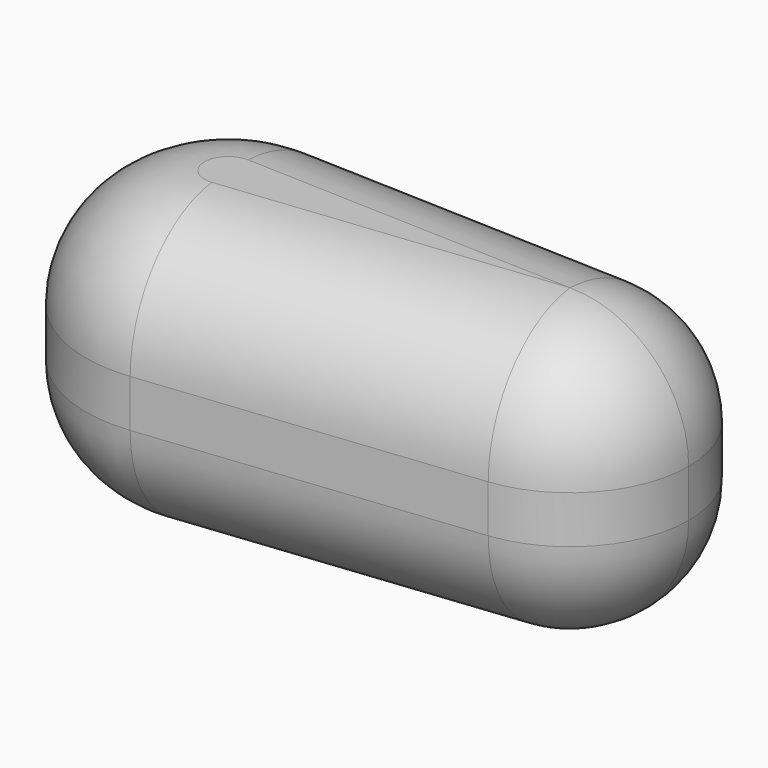
from build123d import *

# Parameters (mm, degrees)
F1_R     = 0.05
F2_DEPTH = 6
F3_DEPTH = 0.05
F4_R     = 5


# Not quite as in the source:
# - a feature names something its author has since deleted; it is built from what else it names


with BuildPart() as f2:
    # F1 (on Top) → F2 (new body, symmetric)
    with BuildSketch(Plane.XY):
        with BuildLine():
            ThreePointArc((-18.3490321939, -11.9655502076), (-14.5272015165, -10.0092257161), (-12.9910685796, -6))
            ThreePointArc((-12.9910685796, -6), (-14.6732359116, -1.8339081802), (-18.7765089299, -0.0038375475))
            ThreePointArc((-18.7765089299, -0.0038375475), (-24.987240828, -6.2142857143), (-18.3490321939, -11.9655502076))
        make_face()
        with Locations((-18.9910685796, -6)):
            Circle(F1_R, mode=Mode.SUBTRACT)
        with BuildLine():
            ThreePointArc((-18.7765089299, -0.0038375475), (-14.6732359116, -1.8339081802), (-12.9910685796, -6))
            ThreePointArc((-12.9910685796, -6), (-14.5272015165, -10.0092257161), (-18.3490321939, -11.9655502076))
            Line((-18.3490321939, -11.9655502076), (-4.4649696785, -10.4712918397))
            ThreePointArc((-4.4649696785, -10.4712918397), (-9.996810207, -5.6785714286), (-4.8212002919, -0.5031979563))
            Line((-4.8212002919, -0.5031979563), (-18.7765089299, -0.0038375475))
        make_face()
        with BuildLine():
            ThreePointArc((0, -5.5), (-1.40180611, -2.0282568169), (-4.8212002919, -0.5031979563))
            ThreePointArc((-4.8212002919, -0.5031979563), (-9.996810207, -5.6785714286), (-4.4649696785, -10.4712918397))
            ThreePointArc((-4.4649696785, -10.4712918397), (-1.2801107807, -8.8410214301), (0, -5.5))
        make_face()
        with Locations((-5, -5.5)):
            Circle(F1_R, mode=Mode.SUBTRACT)
        with Locations((-18.9910685796, -6)):
            Circle(F1_R)
        with Locations((-5, -5.5)):
            Circle(F1_R)
    extrude(amount=F2_DEPTH, both=True)

    # F1 (on Top) → F3 (cut, symmetric)
    with BuildSketch(Plane.XY):
        with Locations((-18.9910685796, -6)):
            Circle(F1_R)
        with Locations((-5, -5.5)):
            Circle(F1_R)
    extrude(amount=F3_DEPTH, both=True, mode=Mode.SUBTRACT)

    # F4
    f4_edges = [f2.edges().sort_by_distance(p)[0] for p in [
        (-24.987241, -6.214286, 6),
        (-11.407001, -11.218421, 6),
        (-0.00319, -5.321429, 6),
        (-11.798855, -0.253518, 6),
        (-24.987241, -6.214286, -6),
        (-11.407001, -11.218421, -6),
        (-0.00319, -5.321429, -6),
        (-11.798855, -0.253518, -6),
    ]]
    fillet(f4_edges, radius=F4_R)


solid = f2.part
